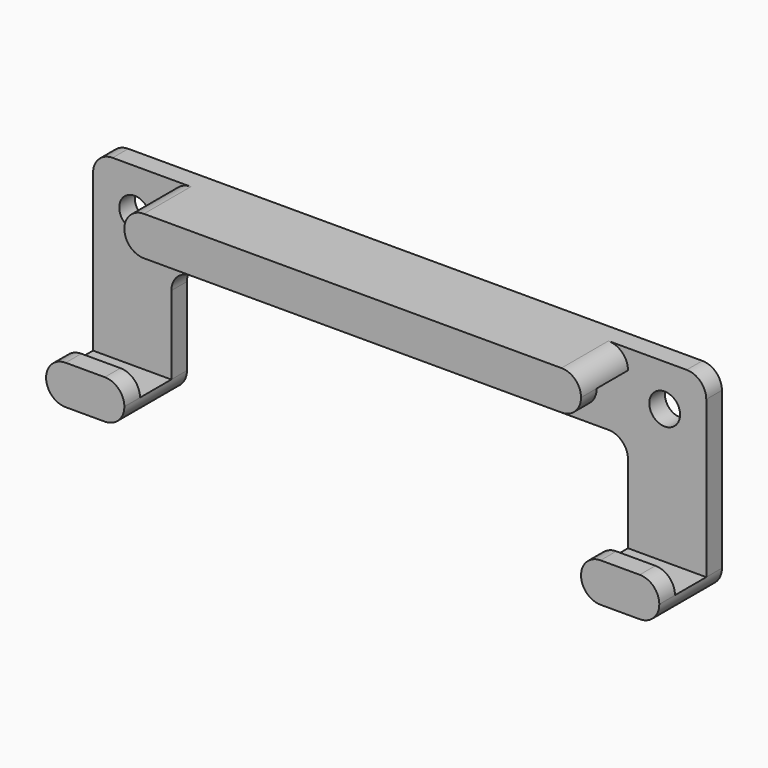
from build123d import *

# Parameters (mm, degrees)
F0_R     = 2.5
F1_DEPTH = 3.175
F2_W     = 12.7
F2_H     = 3.175
F2_W_2   = 74.1
F3_DEPTH = 9.525
F4_W     = 12.7
F4_H     = 3.175
F5_DEPTH = 3.175
F6_W     = 74.1
F6_H     = 3.175
F7_DEPTH = 3.175
F8_R     = 3.17499


# Not quite as in the source:
# - a fillet or chamfer is up to 0.001 mm smaller than in the source, because OpenCascade refuses the exact size


with BuildPart() as f1:
    # F0 (on Front) → F1 (new body)
    with BuildSketch(Plane.XZ):
        Polygon((49.75, -15.875), (49.75, 15.875), (-49.75, 15.875), (-49.75, -15.875), (-37.05, -15.875), (-37.05, 3.175), (37.05, 3.175), (37.05, -15.875), align=None)
        with Locations((-43, 9.125)):
            Circle(F0_R, mode=Mode.SUBTRACT)
        with Locations((43, 9.125)):
            Circle(F0_R, mode=Mode.SUBTRACT)
    extrude(amount=F1_DEPTH)

    # F2 (on face) → F3 (join)
    with BuildSketch(Plane.XZ.offset(3.175)):
        with Locations((-43.4, -14.2875)):
            Rectangle(F2_W, F2_H)
        with Locations((43.4, -14.2875)):
            Rectangle(F2_W, F2_H)
        with Locations((0, 14.2875)):
            Rectangle(F2_W_2, F2_H)
    extrude(amount=F3_DEPTH)

    # F4 (on face) → F5 (join)
    with BuildSketch(Plane.XY.offset(-12.7)):
        with Locations((-43.4, -11.1125)):
            Rectangle(F4_W, F4_H)
        with Locations((43.4, -11.1125)):
            Rectangle(F4_W, F4_H)
    extrude(amount=F5_DEPTH)

    # F6 (on face) → F7 (join)
    with BuildSketch(Plane(origin=(0, 0, 12.7), x_dir=(1, 0, 0), z_dir=(0, 0, -1))):
        with Locations((0, 11.1125)):
            Rectangle(F6_W, F6_H)
    extrude(amount=F7_DEPTH)

    # F8 (radius 3.175 in the source; OpenCascade refuses exactly that, so slightly less here)
    f8_edges = [f1.edges().sort_by_distance(p)[0] for p in [
        (-49.75, -1.5875, 15.875),
        (-49.75, -6.35, -15.875),
        (-37.05, -6.35, -15.875),
        (49.75, -6.35, -15.875),
        (37.05, -6.35, -15.875),
        (49.75, -1.5875, 15.875),
        (37.05, -1.5875, 3.175),
        (-37.05, -1.5875, 3.175),
        (-49.75, -11.1125, -9.525),
        (-37.05, -11.1125, -9.525),
        (49.75, -11.1125, -9.525),
        (37.05, -11.1125, -9.525),
        (-37.05, -7.9375, 15.875),
        (-37.05, -11.1125, 9.525),
        (37.05, -7.9375, 15.875),
        (37.05, -11.1125, 9.525),
    ]]
    fillet(f8_edges, radius=F8_R)


solid = f1.part
